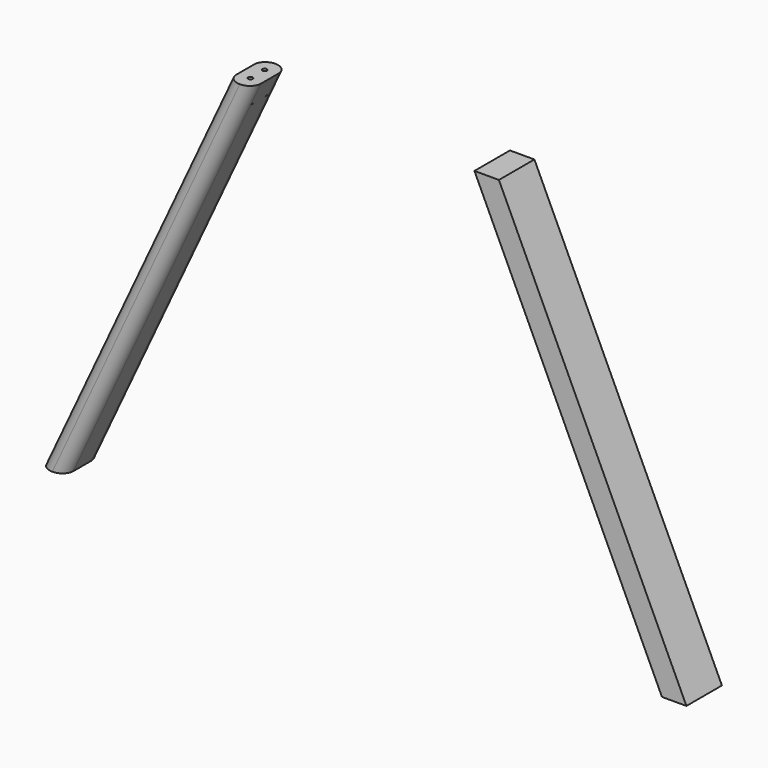
from build123d import *

# Parameters (mm, degrees)
F1_DEPTH = 20
F2_R     = 1
F3_DEPTH = 10
F4_R     = 4.99999


# Not quite as in the source:
# - a fillet or chamfer is up to 0.001 mm smaller than in the source, because OpenCascade refuses the exact size


with BuildPart() as f1:
    # F0 (on Front) → F1 (new body)
    with BuildSketch(Plane.XZ):
        Polygon((586.0166443916, 181.2615574073), (501.4929920435, 0), (512.5267712331, 0), (597.0504235813, 181.2615574073), align=None)
    extrude(amount=F1_DEPTH)

    # F2 (on face) → F3 (cut)
    with BuildSketch(Plane.XY.offset(181.2615574073)):
        with Locations((591.5335339864, -6)):
            Circle(F2_R)
        with Locations((591.5335339864, -14)):
            Circle(F2_R)
    extrude(amount=-F3_DEPTH, mode=Mode.SUBTRACT)

    # F4 (radius 5 in the source; OpenCascade refuses exactly that, so slightly less here)
    f4_edges = [f1.edges().sort_by_distance(p)[0] for p in [
        (543.754818, -20, 90.630779),
        (543.754818, 0, 90.630779),
        (554.788597, -20, 90.630779),
        (554.788597, 0, 90.630779),
    ]]
    fillet(f4_edges, radius=F4_R)


with BuildPart() as f1b:
    # F0 (on Front) → F1, piece 2 (new body)
    with BuildSketch(Plane.XZ):
        Polygon((781.8177731776, 0), (792.8515523672, 0), (708.3279000191, 181.2615574073), (697.2941208294, 181.2615574073), align=None)
    extrude(amount=F1_DEPTH)


solid = Compound([f1.part, f1b.part])
